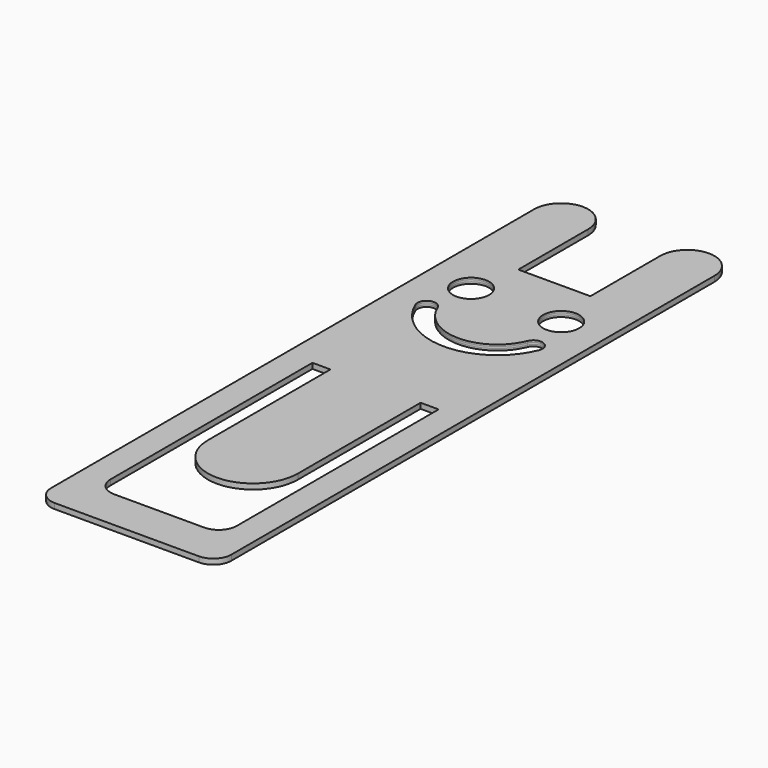
from build123d import *

# Parameters (mm, degrees)
F0_R     = 2
F1_DEPTH = 0.4


# Not quite as in the source:
# - a pattern or mirror of a feature is missing from the dataset's text; its kind, count and spacing are read off the source's solid


with BuildPart() as f1:
    # F0 (on Top) → F1 (new body)
    with BuildSketch(Plane.XY):
        with BuildLine():
            Line((-8, -34.5), (8, -34.5))
            ThreePointArc((8, -34.5), (9.4142135624, -33.9142135624), (10, -32.5))
            Line((10, -32.5), (10, 34.5))
            ThreePointArc((10, 34.5), (7, 37.5), (4, 34.5))
            Line((4, 34.5), (4, 24.8))
            Line((4, 24.8), (-4, 24.8))
            Line((-4, 24.8), (-4, 34.5))
            ThreePointArc((-4, 34.5), (-7, 37.5), (-10, 34.5))
            Line((-10, 34.5), (-10, -32.5))
            ThreePointArc((-10, -32.5), (-9.4142135624, -33.9142135624), (-8, -34.5))
        make_face()
        with BuildLine():
            Line((-7, -28), (-7, 0))
            Line((-7, 0), (-5, 0))
            Line((-5, 0), (5, 0))
            Line((5, 0), (7, 0))
            Line((7, 0), (7, -28))
            ThreePointArc((7, -28), (6.4142135624, -29.4142135624), (5, -30))
            Line((5, -30), (-5, -30))
            ThreePointArc((-5, -30), (-6.4142135624, -29.4142135624), (-7, -28))
        make_face(mode=Mode.SUBTRACT)
        with Locations((-5, 19.5)):
            Circle(F0_R, mode=Mode.SUBTRACT)
        with BuildLine():
            ThreePointArc((-5, 14.8603921946), (0, 11.5), (5, 14.8603921946))
            ThreePointArc((5, 14.8603921946), (6.3036310751, 15.4086129713), (6.8518518519, 14.1049818963))
            ThreePointArc((6.8518518519, 14.1049818963), (0, 9.5), (-6.8518518519, 14.1049818963))
            ThreePointArc((-6.8518518519, 14.1049818963), (-6.3036310751, 15.4086129713), (-5, 14.8603921946))
        make_face(mode=Mode.SUBTRACT)
        with Locations((5, 19.5)):
            Circle(F0_R, mode=Mode.SUBTRACT)
        with BuildLine():
            Line((5, 0), (-5, 0))
            Line((-5, 0), (-5, -17))
            ThreePointArc((-5, -17), (0, -22), (5, -17))
            Line((5, -17), (5, 0))
        make_face()
    extrude(amount=F1_DEPTH)

    # F1_copies: F1 across plane


with BuildPart() as f1_1:
    add(f1.part)
    add(f1.part.mirror(Plane.XY.offset(0.3)))


solid = f1_1.part
